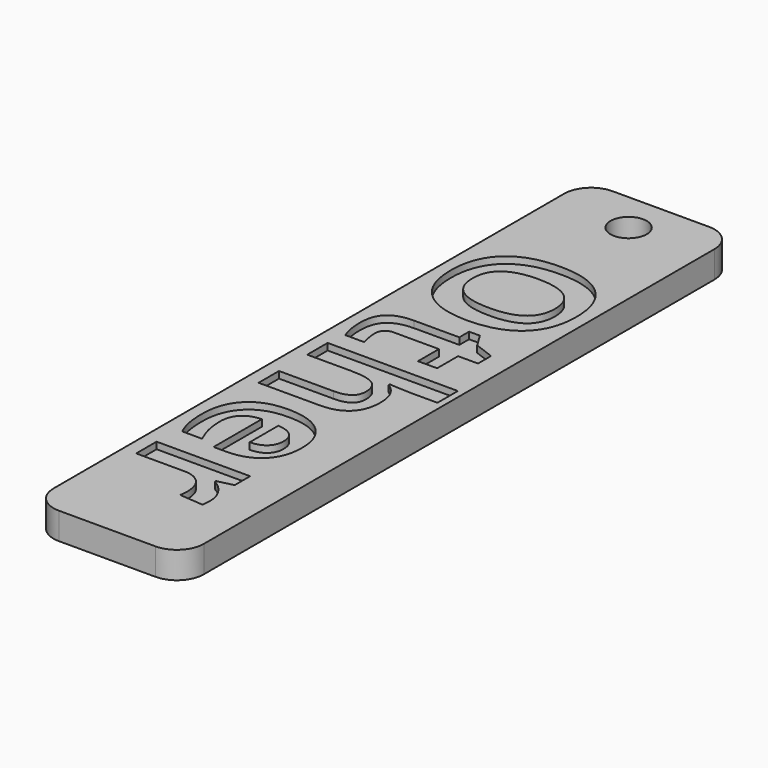
from build123d import *

# Parameters (mm, degrees)
F0_W         = 11.2
F0_H         = 51.6
F0_R         = 1.35
F0_TEXT_SIZE = 12.7777777778
F1_DEPTH     = 2
F2_DEPTH     = 0.5
F3_R         = 2


# Not quite as in the source:
# - Text() gives the source's letters only with a copy of the font that has no kerning and outlines rounded to 1/6400 em; it was checked with that copy


with BuildPart() as f1:
    # F0 (on Top) → F1 (new body)
    with BuildSketch(Plane.XY):
        with Locations((-43.6647401989, 47.9276468577)):
            Rectangle(F0_W, F0_H)
        with BuildLine():
            add(Edge.make_bspline(
                [(-41.5174745739, 29.7870652605), (-41.1590978377, 29.23502533), (-41.1590978377, 28.5861538022)],
                knots=[0, 0, 0, 1, 1, 1], degree=2))
            add(Edge.make_bspline(
                [(-41.1590978377, 28.5861538022), (-41.1590978377, 28.1988274133), (-41.2150006155, 27.9432718577)],
                knots=[0, 0, 0, 1, 1, 1], degree=2))
            Line((-41.2150006155, 27.9432718577), (-42.9978999211, 28.0870218577))
            add(Edge.make_bspline(
                [(-42.9978999211, 28.0870218577), (-42.93600756, 28.31861908), (-42.93600756, 28.6480461633)],
                knots=[0, 0, 0, 1, 1, 1], degree=2))
            add(Edge.make_bspline(
                [(-42.93600756, 28.6480461633), (-42.93600756, 29.55846283), (-43.4041933239, 30.0675774133)],
                knots=[0, 0, 0, 1, 1, 1], degree=2))
            add(Edge.make_bspline(
                [(-43.4041933239, 30.0675774133), (-43.8723790877, 30.5766919966), (-44.71491381, 30.5766919966)],
                knots=[0, 0, 0, 1, 1, 1], degree=2))
            Line((-44.71491381, 30.5766919966), (-48.2647401989, 30.5766919966))
            Line((-48.2647401989, 30.5766919966), (-48.2647401989, 32.4793829688))
            Line((-48.2647401989, 32.4793829688), (-41.2888721433, 32.4793829688))
            Line((-41.2888721433, 32.4793829688), (-41.2888721433, 31.0378899133))
            Line((-41.2888721433, 31.0378899133), (-42.4628304766, 30.7563794966))
            Line((-42.4628304766, 30.7563794966), (-42.4628304766, 30.6645392188))
            add(Edge.make_bspline(
                [(-42.4628304766, 30.6645392188), (-41.87585131, 30.3391051911), (-41.5174745739, 29.7870652605)],
                knots=[0, 0, 0, 1, 1, 1], degree=2))
        make_face(mode=Mode.SUBTRACT)
        with BuildLine():
            add(Edge.make_bspline(
                [(-48.2687332544, 35.4861538022), (-48.3905214489, 36.0531676911), (-48.3905214489, 36.87174408)],
                knots=[0, 0, 0, 1, 1, 1], degree=2))
            add(Edge.make_bspline(
                [(-48.3905214489, 36.87174408), (-48.3905214489, 38.5548169966), (-47.4601395044, 39.5031676911)],
                knots=[0, 0, 0, 1, 1, 1], degree=2))
            add(Edge.make_bspline(
                [(-47.4601395044, 39.5031676911), (-46.52975756, 40.4515183855), (-44.8267193655, 40.4515183855)],
                knots=[0, 0, 0, 1, 1, 1], degree=2))
            add(Edge.make_bspline(
                [(-44.8267193655, 40.4515183855), (-43.0737679766, 40.4515183855), (-42.1164329072, 39.5750426911)],
                knots=[0, 0, 0, 1, 1, 1], degree=2))
            add(Edge.make_bspline(
                [(-42.1164329072, 39.5750426911), (-41.1590978377, 38.6985669966), (-41.1590978377, 37.1512579688)],
                knots=[0, 0, 0, 1, 1, 1], degree=2))
            add(Edge.make_bspline(
                [(-41.1590978377, 37.1512579688), (-41.1590978377, 35.6738274133), (-42.0006342961, 34.850259705)],
                knots=[0, 0, 0, 1, 1, 1], degree=2))
            add(Edge.make_bspline(
                [(-42.0006342961, 34.850259705), (-42.8421707544, 34.0266919966), (-44.3275874211, 34.0266919966)],
                knots=[0, 0, 0, 1, 1, 1], degree=2))
            Line((-44.3275874211, 34.0266919966), (-45.2519797822, 34.0266919966))
            Line((-45.2519797822, 34.0266919966), (-45.2519797822, 38.52486908))
            add(Edge.make_bspline(
                [(-45.2519797822, 38.52486908), (-46.06257006, 38.4929246355), (-46.5177783933, 38.0437058855)],
                knots=[0, 0, 0, 1, 1, 1], degree=2))
            add(Edge.make_bspline(
                [(-46.5177783933, 38.0437058855), (-46.9729867266, 37.5944871355), (-46.9729867266, 36.7838968577)],
                knots=[0, 0, 0, 1, 1, 1], degree=2))
            add(Edge.make_bspline(
                [(-46.9729867266, 36.7838968577), (-46.9729867266, 36.15299408), (-46.8422141572, 35.5919697744)],
                knots=[0, 0, 0, 1, 1, 1], degree=2))
            add(Edge.make_bspline(
                [(-46.8422141572, 35.5919697744), (-46.7114415877, 35.0309454688), (-46.4239415877, 34.4200079688)],
                knots=[0, 0, 0, 1, 1, 1], degree=2))
            Line((-46.4239415877, 34.4200079688), (-47.8973790877, 34.4200079688))
            add(Edge.make_bspline(
                [(-47.8973790877, 34.4200079688), (-48.14694506, 34.9191399133), (-48.2687332544, 35.4861538022)],
                knots=[0, 0, 0, 1, 1, 1], degree=2))
        make_face(mode=Mode.SUBTRACT)
        with BuildLine():
            Line((-43.7166499211, 41.9868482466), (-48.2647401989, 41.9868482466))
            Line((-48.2647401989, 41.9868482466), (-48.2647401989, 43.8895392188))
            Line((-48.2647401989, 43.8895392188), (-44.1898270044, 43.8895392188))
            add(Edge.make_bspline(
                [(-44.1898270044, 43.8895392188), (-42.6804520044, 43.8895392188), (-42.6804520044, 45.0135843577)],
                knots=[0, 0, 0, 1, 1, 1], degree=2))
            add(Edge.make_bspline(
                [(-42.6804520044, 45.0135843577), (-42.6804520044, 45.8121954688), (-43.22350756, 46.1675774133)],
                knots=[0, 0, 0, 1, 1, 1], degree=2))
            add(Edge.make_bspline(
                [(-43.22350756, 46.1675774133), (-43.7665631155, 46.5229593577), (-44.9824485322, 46.5229593577)],
                knots=[0, 0, 0, 1, 1, 1], degree=2))
            Line((-44.9824485322, 46.5229593577), (-48.2647401989, 46.5229593577))
            Line((-48.2647401989, 46.5229593577), (-48.2647401989, 48.42565033))
            Line((-48.2647401989, 48.42565033), (-38.5556256155, 48.42565033))
            Line((-38.5556256155, 48.42565033), (-38.5556256155, 46.5229593577))
            Line((-38.5556256155, 46.5229593577), (-40.5341846433, 46.5229593577))
            add(Edge.make_bspline(
                [(-40.5341846433, 46.5229593577), (-40.7657818655, 46.5229593577), (-41.6202957544, 46.5668829688)],
                knots=[0, 0, 0, 1, 1, 1], degree=2))
            Line((-41.6202957544, 46.5668829688), (-42.18132006, 46.61080658))
            Line((-42.18132006, 46.61080658), (-42.18132006, 46.5109801911))
            add(Edge.make_bspline(
                [(-42.18132006, 46.5109801911), (-41.1590978377, 45.87408783), (-41.1590978377, 44.4884975522)],
                knots=[0, 0, 0, 1, 1, 1], degree=2))
            add(Edge.make_bspline(
                [(-41.1590978377, 44.4884975522), (-41.1590978377, 43.2586364411), (-41.8199485322, 42.6227423438)],
                knots=[0, 0, 0, 1, 1, 1], degree=2))
            add(Edge.make_bspline(
                [(-41.8199485322, 42.6227423438), (-42.4807992266, 41.9868482466), (-43.7166499211, 41.9868482466)],
                knots=[0, 0, 0, 1, 1, 1], degree=2))
        make_face(mode=Mode.SUBTRACT)
        with BuildLine():
            add(Edge.make_bspline(
                [(-46.6794971433, 51.6360669966), (-46.8731603377, 51.40846283), (-46.8731603377, 51.0331156077)],
                knots=[0, 0, 0, 1, 1, 1], degree=2))
            add(Edge.make_bspline(
                [(-46.8731603377, 51.0331156077), (-46.8731603377, 50.5339836633), (-46.65553881, 49.8351989411)],
                knots=[0, 0, 0, 1, 1, 1], degree=2))
            Line((-46.65553881, 49.8351989411), (-48.0710770044, 49.8351989411))
            add(Edge.make_bspline(
                [(-48.0710770044, 49.8351989411), (-48.3905214489, 50.54596283), (-48.3905214489, 51.5821607466)],
                knots=[0, 0, 0, 1, 1, 1], degree=2))
            add(Edge.make_bspline(
                [(-48.3905214489, 51.5821607466), (-48.3905214489, 52.7241746355), (-47.8125266572, 53.2452683855)],
                knots=[0, 0, 0, 1, 1, 1], degree=2))
            add(Edge.make_bspline(
                [(-47.8125266572, 53.2452683855), (-47.2345318655, 53.7663621355), (-46.08053881, 53.7663621355)],
                knots=[0, 0, 0, 1, 1, 1], degree=2))
            Line((-46.08053881, 53.7663621355), (-42.7183860322, 53.7663621355))
            Line((-42.7183860322, 53.7663621355), (-42.7183860322, 54.6767788022))
            Line((-42.7183860322, 54.6767788022), (-41.9137853377, 54.6767788022))
            Line((-41.9137853377, 54.6767788022), (-41.2768929766, 53.6286017188))
            Line((-41.2768929766, 53.6286017188), (-39.8034554766, 53.07955658))
            Line((-39.8034554766, 53.07955658), (-39.8034554766, 51.8636711633))
            Line((-39.8034554766, 51.8636711633), (-41.2888721433, 51.8636711633))
            Line((-41.2888721433, 51.8636711633), (-41.2888721433, 49.9110669966))
            Line((-41.2888721433, 49.9110669966), (-42.7183860322, 49.9110669966))
            Line((-42.7183860322, 49.9110669966), (-42.7183860322, 51.8636711633))
            Line((-42.7183860322, 51.8636711633), (-46.08053881, 51.8636711633))
            add(Edge.make_bspline(
                [(-46.08053881, 51.8636711633), (-46.4858339489, 51.8636711633), (-46.6794971433, 51.6360669966)],
                knots=[0, 0, 0, 1, 1, 1], degree=2))
        make_face(mode=Mode.SUBTRACT)
        with BuildLine():
            add(Edge.make_bspline(
                [(-40.2097488794, 56.8270392188), (-41.4206429766, 55.7129767188), (-43.69069506, 55.7129767188)],
                knots=[0, 0, 0, 1, 1, 1], degree=2))
            add(Edge.make_bspline(
                [(-43.69069506, 55.7129767188), (-45.9567540877, 55.7129767188), (-47.1736377683, 56.8360235938)],
                knots=[0, 0, 0, 1, 1, 1], degree=2))
            add(Edge.make_bspline(
                [(-47.1736377683, 56.8360235938), (-48.3905214489, 57.9590704688), (-48.3905214489, 60.0554246355)],
                knots=[0, 0, 0, 1, 1, 1], degree=2))
            add(Edge.make_bspline(
                [(-48.3905214489, 60.0554246355), (-48.3905214489, 62.1517788022), (-47.1736377683, 63.2748256772)],
                knots=[0, 0, 0, 1, 1, 1], degree=2))
            add(Edge.make_bspline(
                [(-47.1736377683, 63.2748256772), (-45.9567540877, 64.3978725522), (-43.6787158933, 64.3978725522)],
                knots=[0, 0, 0, 1, 1, 1], degree=2))
            add(Edge.make_bspline(
                [(-43.6787158933, 64.3978725522), (-41.4006776989, 64.3978725522), (-40.1997662405, 63.2718308855)],
                knots=[0, 0, 0, 1, 1, 1], degree=2))
            add(Edge.make_bspline(
                [(-40.1997662405, 63.2718308855), (-38.9988547822, 62.1457892188), (-38.9988547822, 60.0434454688)],
                knots=[0, 0, 0, 1, 1, 1], degree=2))
            add(Edge.make_bspline(
                [(-38.9988547822, 60.0434454688), (-38.9988547822, 57.9411017188), (-40.2097488794, 56.8270392188)],
                knots=[0, 0, 0, 1, 1, 1], degree=2))
        make_face(mode=Mode.SUBTRACT)
        with Locations((-43.6647401989, 70.7276468577)):
            Circle(F0_R, mode=Mode.SUBTRACT)
        with BuildLine():
            add(Edge.make_bspline(
                [(-41.3867020044, 61.7834194272), (-42.16335131, 62.36940033), (-43.69069506, 62.36940033)],
                knots=[0, 0, 0, 1, 1, 1], degree=2))
            add(Edge.make_bspline(
                [(-43.69069506, 62.36940033), (-45.2200353377, 62.36940033), (-45.9936898516, 61.7894090105)],
                knots=[0, 0, 0, 1, 1, 1], degree=2))
            add(Edge.make_bspline(
                [(-45.9936898516, 61.7894090105), (-46.7673443655, 61.2094176911), (-46.7673443655, 60.0554246355)],
                knots=[0, 0, 0, 1, 1, 1], degree=2))
            add(Edge.make_bspline(
                [(-46.7673443655, 60.0554246355), (-46.7673443655, 57.7414489411), (-43.69069506, 57.7414489411)],
                knots=[0, 0, 0, 1, 1, 1], degree=2))
            add(Edge.make_bspline(
                [(-43.69069506, 57.7414489411), (-40.6100526989, 57.7414489411), (-40.6100526989, 60.0434454688)],
                knots=[0, 0, 0, 1, 1, 1], degree=2))
            add(Edge.make_bspline(
                [(-40.6100526989, 60.0434454688), (-40.6100526989, 61.1974385244), (-41.3867020044, 61.7834194272)],
                knots=[0, 0, 0, 1, 1, 1], degree=2))
        make_face()
        with Locations(Location((-48.2647401989, 65.1405808855), (0, 0, -90))):
            Text('Other', F0_TEXT_SIZE, font='Open Sans', font_style=FontStyle.BOLD, text_align=(TextAlign.LEFT, TextAlign.BOTTOM))
        with BuildLine():
            add(Edge.make_bspline(
                [(-42.8960770044, 36.1789489411), (-42.5127436711, 36.5343308855), (-42.5127436711, 37.1392788022)],
                knots=[0, 0, 0, 1, 1, 1], degree=2))
            add(Edge.make_bspline(
                [(-42.5127436711, 37.1392788022), (-42.5127436711, 37.7442267188), (-42.8960770044, 38.0876294966)],
                knots=[0, 0, 0, 1, 1, 1], degree=2))
            add(Edge.make_bspline(
                [(-42.8960770044, 38.0876294966), (-43.2794103377, 38.4310322744), (-43.9841846433, 38.4809454688)],
                knots=[0, 0, 0, 1, 1, 1], degree=2))
            Line((-43.9841846433, 38.4809454688), (-43.9841846433, 35.8095913022))
            add(Edge.make_bspline(
                [(-43.9841846433, 35.8095913022), (-43.2794103377, 35.8235669966), (-42.8960770044, 36.1789489411)],
                knots=[0, 0, 0, 1, 1, 1], degree=2))
        make_face()
    extrude(amount=-F1_DEPTH)

    # F0 (on Top) → F2 (cut)
    with BuildSketch(Plane.XY):
        with Locations(Location((-48.2647401989, 65.1405808855), (0, 0, -90))):
            Text('Other', F0_TEXT_SIZE, font='Open Sans', font_style=FontStyle.BOLD, text_align=(TextAlign.LEFT, TextAlign.BOTTOM))
    extrude(amount=-F2_DEPTH, mode=Mode.SUBTRACT)

    # F3
    f3_edges = [f1.edges().sort_by_distance(p)[0] for p in [
        (-49.26474, 73.727647, -1),
        (-38.06474, 73.727647, -1),
        (-38.06474, 22.127647, -1),
        (-49.26474, 22.127647, -1),
    ]]
    fillet(f3_edges, radius=F3_R)


solid = f1.part
